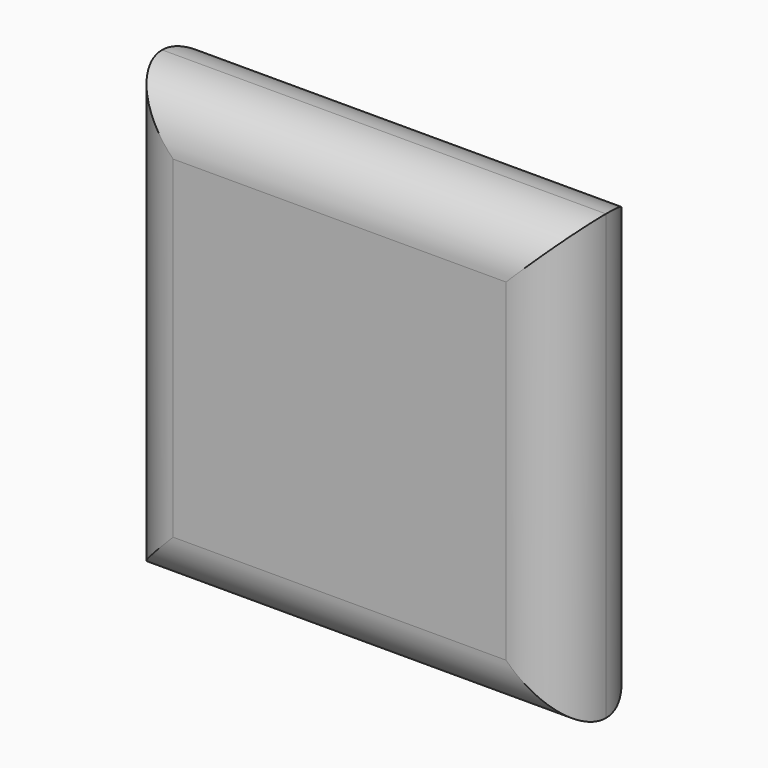
from build123d import *

# Parameters (mm, degrees)
F0_W     = 101.6
F0_H     = 101.6
F1_DEPTH = 25.4
F2_R     = 12.69999


# Not quite as in the source:
# - a fillet or chamfer is up to 0.001 mm smaller than in the source, because OpenCascade refuses the exact size


with BuildPart() as f1:
    # F0 (on Front) → F1 (new body)
    with BuildSketch(Plane.XZ):
        with Locations((12.5491575718, -14.5562545776)):
            Rectangle(F0_W, F0_H)
    extrude(amount=F1_DEPTH)

    # F2 (radius 12.7 in the source; OpenCascade refuses exactly that, so slightly less here)
    f2_edges = [f1.edges().sort_by_distance(p)[0] for p in [
        (12.549158, 0, -65.356255),
        (63.349158, 0, -14.556255),
        (12.549158, 0, 36.243745),
        (-38.250842, 0, -14.556255),
        (12.549158, -25.4, -65.356255),
        (63.349158, -25.4, -14.556255),
        (12.549158, -25.4, 36.243745),
        (-38.250842, -25.4, -14.556255),
    ]]
    fillet(f2_edges, radius=F2_R)


solid = f1.part
